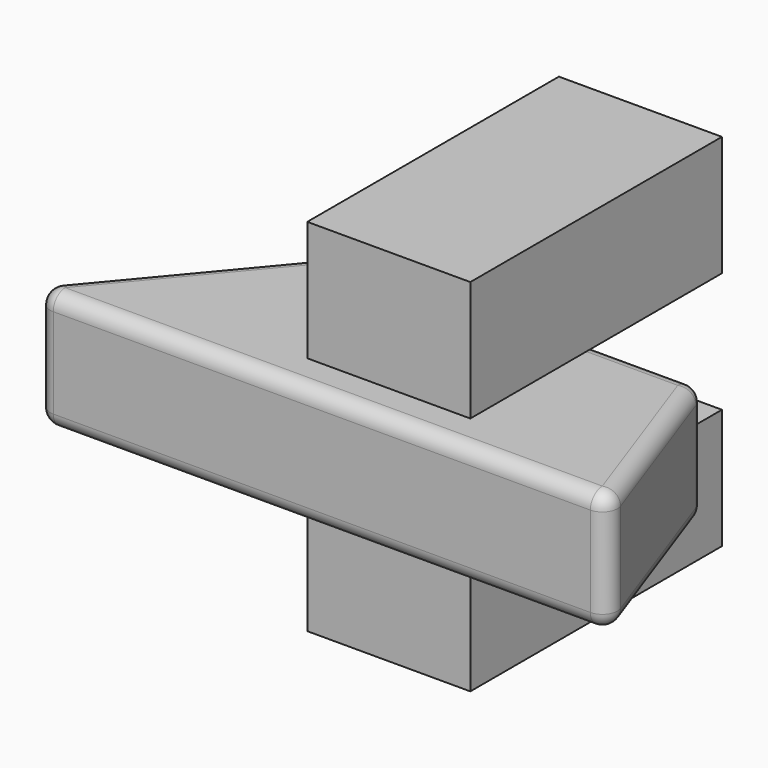
from build123d import *

# Parameters (mm, degrees)
F1_DEPTH = 25.4
F2_R     = 6.35
F3_R     = 15.9134591768
F4_DEPTH = 50.801
F5_W     = 68.9585166983
F5_H     = 133.0089531839
F6_DEPTH = 50.8
F8_R     = 15.9134591768
F9_DEPTH = 50.8


with BuildPart() as f1:
    # F0 (on Top) → F1 (new body, symmetric)
    with BuildSketch(Plane.XY):
        Polygon((-39.645280689, 27.3465514183), (-110.2543845773, -57.1528710425), (139.4819170237, -57.1528710425), (109.386228025, 27.3465514183), align=None)
    extrude(amount=F1_DEPTH, both=True)

    # F2
    f2_edges = [f1.edges().sort_by_distance(p)[0] for p in [
        (109.386228, 27.346551, 0),
        (34.870474, 27.346551, -25.4),
        (-39.645281, 27.346551, 0),
        (34.870474, 27.346551, 25.4),
        (-74.949833, -14.90316, -25.4),
        (-110.254385, -57.152871, 0),
        (-74.949833, -14.90316, 25.4),
        (139.481917, -57.152871, 0),
        (124.434073, -14.90316, -25.4),
        (124.434073, -14.90316, 25.4),
        (14.613766, -57.152871, -25.4),
        (14.613766, -57.152871, 25.4),
    ]]
    fillet(f2_edges, radius=F2_R)

    # F3 (on face) → F4 (cut, through all)
    with BuildSketch(Plane.XY.offset(25.4)):
        with Locations((29.4188149273, -14.7804608569)):
            Circle(F3_R)
    extrude(amount=-F4_DEPTH, mode=Mode.SUBTRACT)


with BuildPart() as f6:
    # F5 (on face) → F6 (new body)
    with BuildSketch(Plane.XY.offset(25.4)):
        with Locations((31.7501595709, 26.2020025402)):
            Rectangle(F5_W, F5_H)
    extrude(amount=F6_DEPTH)


with BuildPart() as f7_1:
    # F7: instance of F6
    add(f6.part.mirror(Plane.XY))


with BuildPart() as f6_1:
    add(f6.part)

    add(f7_1.part)  # F9 merges F7_1
    # F8 (on face) → F9 (join, through all)
    with BuildSketch(Plane.XY.offset(-25.4)):
        with Locations((29.4188149273, -14.7804608569)):
            Circle(F8_R)
    extrude(amount=F9_DEPTH)


solid = Compound([f1.part, f6_1.part])
